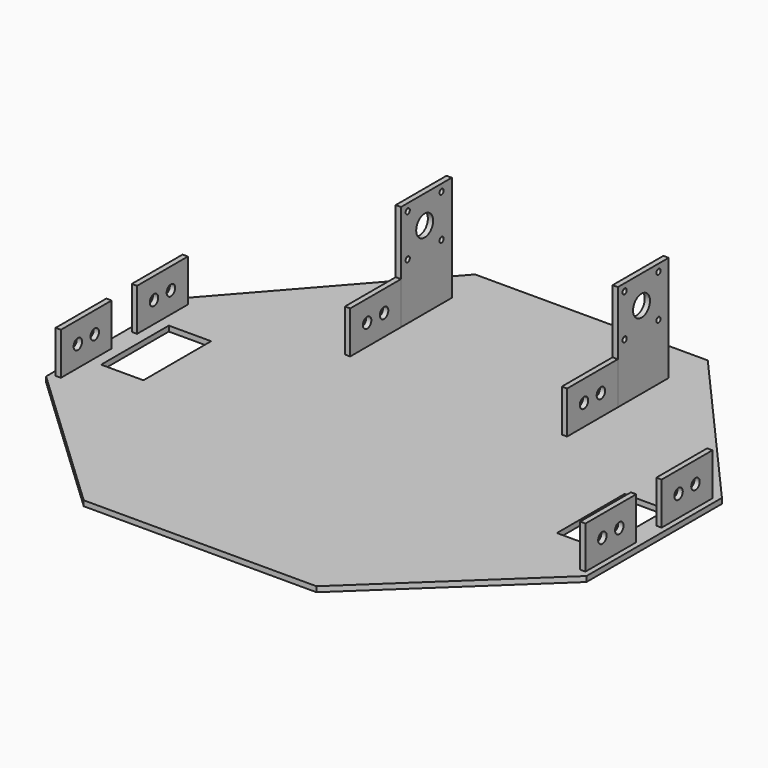
from build123d import *

# Parameters (mm, degrees)
F1_DEPTH  = 3.175
F2_W      = 3.175
F2_H      = 38.1
F3_DEPTH  = 25.4
F4_R      = 3.175
F5_DEPTH  = 381
F2_W_2    = 25.4
F2_H_2    = 50.8
F6_DEPTH  = 25.4
F7_DEPTH  = 63.5
F8_R      = 6.35
F9_DEPTH  = 177.8
F11_DEPTH = 304.8
F12_DEPTH = 25.4
F13_DEPTH = 254


# Not quite as in the source:
# - ends of sketch curves that miss each other by under 0.0002 mm in the source are joined
# - a feature names something its author has since deleted; it is built from what else it names


with BuildPart() as f1:
    # F0 (on Top) → F1 (new body)
    with BuildSketch(Plane.XY):
        Polygon((-252.9524413709, 74.0429753427), (-252.9524413709, -27.5570246573), (-160.6017448068, -114.7370042634), (-20.9017448068, -114.7370042634), (71.4489517573, -27.5570246573), (71.4489517573, 74.0429753427), (-20.9017448068, 178.8639600935), (-160.6017448068, 178.8639600935), align=None)
    extrude(amount=F1_DEPTH)

    # F2 (on face) → F3 (join)
    with BuildSketch(Plane.XY.offset(3.175)):
        with Locations((-248.1899413709, 51.8179753427)):
            Rectangle(F2_W, F2_H)
        with Locations((-248.1899413709, -5.3320246573)):
            Rectangle(F2_W, F2_H)
        with Locations((-155.8392448068, 96.3139587522)):
            Rectangle(F2_W, F2_H)
        with Locations((-25.6642448068, 96.3139587522)):
            Rectangle(F2_W, F2_H)
        with Locations((66.6864517573, 51.8179753427)):
            Rectangle(F2_W, F2_H)
        with Locations((66.6864517573, -5.3320246573)):
            Rectangle(F2_W, F2_H)
    extrude(amount=F3_DEPTH)

    # F4 (on Right) → F5 (cut, symmetric)
    with BuildSketch(Plane.YZ):
        with Locations((-11.6820246573, 15.875)):
            Circle(F4_R)
        with Locations((1.0179753427, 15.875)):
            Circle(F4_R)
        with Locations((45.4679753427, 15.875)):
            Circle(F4_R)
        with Locations((58.1679753427, 15.875)):
            Circle(F4_R)
        with Locations((89.9639587522, 15.875)):
            Circle(F4_R)
        with Locations((102.6639587522, 15.875)):
            Circle(F4_R)
    extrude(amount=F5_DEPTH, both=True, mode=Mode.SUBTRACT)

    # F2 (on face) → F6 (cut)
    with BuildSketch(Plane.XY.offset(3.175)):
        with Locations((-227.5524413709, 23.2429753427)):
            Rectangle(F2_W_2, F2_H_2)
        with Locations((46.0489517573, 23.2429753427)):
            Rectangle(F2_W_2, F2_H_2)
    extrude(amount=-F6_DEPTH, mode=Mode.SUBTRACT)

    # F2 (on face) → F7 (join)
    with BuildSketch(Plane.XY.offset(3.175)):
        with Locations((-155.8392446995, 134.4139587522)):
            Rectangle(F2_W, F2_H)
        with Locations((-25.6642446429, 134.4139587522)):
            Rectangle(F2_W, F2_H)
    extrude(amount=F7_DEPTH)

    # F8 (on face) + F4 (on Right) → F9 (cut, symmetric)
    with BuildSketch(Plane.YZ.offset(-24.0767446429)):
        with Locations((133.1326216459, 49.6721826494)):
            Circle(F8_R)
    with BuildSketch(Plane.YZ):
        with Locations((89.9639587522, 15.875)):
            Circle(F4_R)
        with Locations((102.6639587522, 15.875)):
            Circle(F4_R)
    extrude(amount=F9_DEPTH, both=True, mode=Mode.SUBTRACT)

    # F10 (on face) → F11 (cut)
    with BuildSketch(Plane.YZ.offset(-24.0767446429)):
        with BuildLine():
            ThreePointArc((122.0201216459, 62.3721826494), (119.3100896308, 63.4947146645), (120.4326216459, 60.7846826494))
            Line((120.4326216459, 60.7846826494), (120.4326216459, 62.3721826494))
            Line((120.4326216459, 62.3721826494), (122.0201216459, 62.3721826494))
        make_face()
        with BuildLine():
            Line((145.8326216459, 62.3721826494), (145.8326216459, 60.7846826494))
            ThreePointArc((145.8326216459, 60.7846826494), (146.9551536611, 61.2496506342), (147.4201216459, 62.3721826494))
            ThreePointArc((147.4201216459, 62.3721826494), (145.8326216459, 63.9596826494), (144.2451216459, 62.3721826494))
            Line((144.2451216459, 62.3721826494), (145.8326216459, 62.3721826494))
        make_face()
        with BuildLine():
            Line((145.8326216459, 36.9721826494), (144.2451216459, 36.9721826494))
            ThreePointArc((144.2451216459, 36.9721826494), (145.8326216459, 35.3846826494), (147.4201216459, 36.9721826494))
            ThreePointArc((147.4201216459, 36.9721826494), (146.9551536611, 38.0947146645), (145.8326216459, 38.5596826494))
            Line((145.8326216459, 38.5596826494), (145.8326216459, 36.9721826494))
        make_face()
        with BuildLine():
            ThreePointArc((120.4326216459, 38.5596826494), (119.3100896308, 35.8496506342), (122.0201216459, 36.9721826494))
            Line((122.0201216459, 36.9721826494), (120.4326216459, 36.9721826494))
            Line((120.4326216459, 36.9721826494), (120.4326216459, 38.5596826494))
        make_face()
        with BuildLine():
            Line((120.4326216459, 36.9721826494), (122.0201216459, 36.9721826494))
            ThreePointArc((122.0201216459, 36.9721826494), (121.5551536611, 38.0947146645), (120.4326216459, 38.5596826494))
            Line((120.4326216459, 38.5596826494), (120.4326216459, 36.9721826494))
        make_face()
        with BuildLine():
            Line((120.4326216459, 62.3721826494), (120.4326216459, 60.7846826494))
            ThreePointArc((120.4326216459, 60.7846826494), (121.5551536611, 61.2496506342), (122.0201216459, 62.3721826494))
            Line((122.0201216459, 62.3721826494), (120.4326216459, 62.3721826494))
        make_face()
        with BuildLine():
            ThreePointArc((144.2451216459, 62.3721826494), (144.7100896308, 61.2496506342), (145.8326216459, 60.7846826494))
            Line((145.8326216459, 60.7846826494), (145.8326216459, 62.3721826494))
            Line((145.8326216459, 62.3721826494), (144.2451216459, 62.3721826494))
        make_face()
        with BuildLine():
            ThreePointArc((145.8326216459, 38.5596826494), (144.7100896308, 38.0947146645), (144.2451216459, 36.9721826494))
            Line((144.2451216459, 36.9721826494), (145.8326216459, 36.9721826494))
            Line((145.8326216459, 36.9721826494), (145.8326216459, 38.5596826494))
        make_face()
    extrude(amount=-F11_DEPTH, mode=Mode.SUBTRACT)

    # F2 (on face) → F12 (join)
    with BuildSketch(Plane.XY.offset(3.175)):
        with Locations((-25.6642448068, 96.3139587522)):
            Rectangle(F2_W, F2_H)
        with Locations((-155.8392448068, 96.3139587522)):
            Rectangle(F2_W, F2_H)
    extrude(amount=F12_DEPTH)

    # F4 (on Right) → F13 (cut)
    with BuildSketch(Plane.YZ):
        with Locations((102.6639587522, 15.875)):
            Circle(F4_R)
        with Locations((89.9639587522, 15.875)):
            Circle(F4_R)
    extrude(amount=-F13_DEPTH, mode=Mode.SUBTRACT)


solid = f1.part
